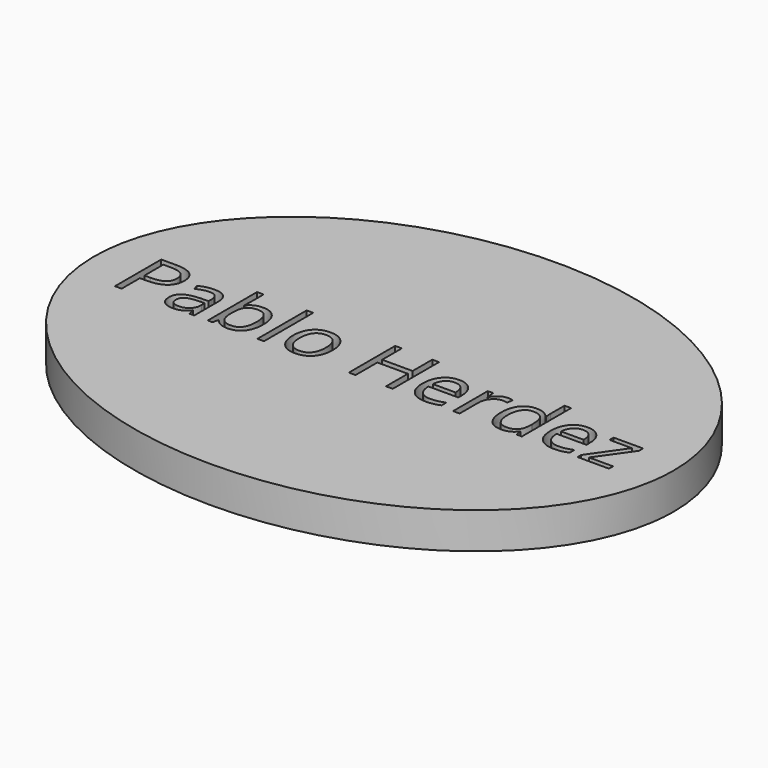
from build123d import *

# Parameters (mm, degrees)
F1_DEPTH     = 6.35
F2_TEXT_SIZE = 14.1966714075
F3_DEPTH     = 3.175


# Not quite as in the source:
# - Text() gives the source's letters only with a copy of the font that has no kerning and outlines rounded to 1/6400 em; it was checked with that copy


with BuildPart() as f1:
    # F0 (on Top) → F1 (new body)
    with BuildSketch(Plane.XY):
        with BuildLine():
            add(Edge.make_bspline(
                [(50.8, 0), (50.8, 65.9911357684), (-25.4, 32.9955678842), (-101.6, 0), (-25.4, -32.9955678842), (50.8, -65.9911357684), (50.8, 0)],
                knots=[0, 0, 0, 2.0943951024, 2.0943951024, 4.1887902048, 4.1887902048, 6.2831853072, 6.2831853072, 6.2831853072], degree=2, weights=[1, 0.5, 1, 0.5, 1, 0.5, 1]))
        make_face()
    extrude(amount=F1_DEPTH)

    # F2 (on face) → F3 (cut)
    with BuildSketch(Plane.XY.offset(6.35)):
        with Locations((-44.45, -5.1108017067)):
            Text('Pablo Herdez', F2_TEXT_SIZE, font='Open Sans', text_align=(TextAlign.LEFT, TextAlign.BOTTOM))
    extrude(amount=-F3_DEPTH, mode=Mode.SUBTRACT)


solid = f1.part
